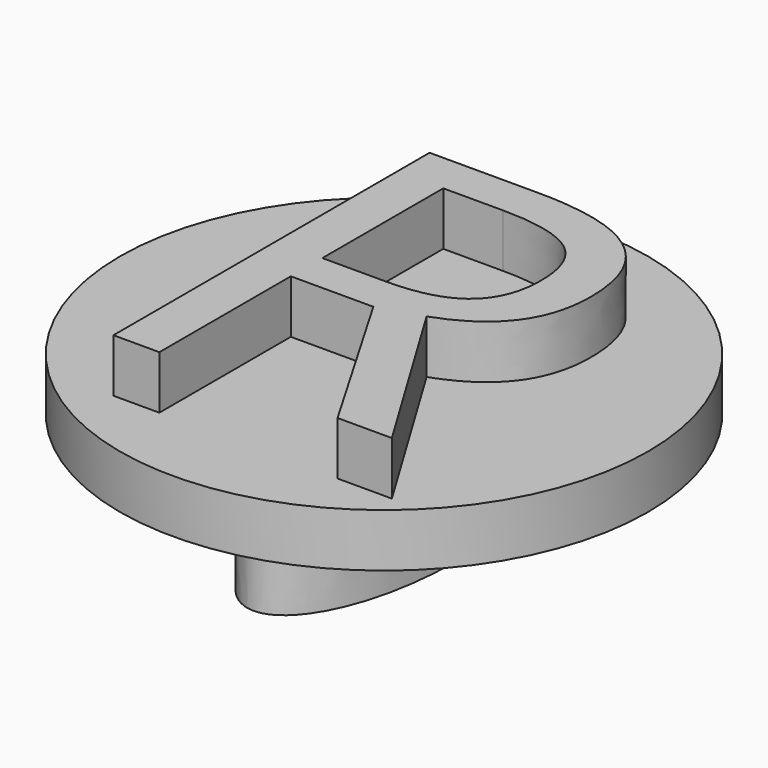
from build123d import *

# Parameters (mm, degrees)
F0_TEXT_SIZE = 26.3821948061
F1_DEPTH     = 5.08
F2_R         = 12.5880099823
F3_DEPTH     = 2.54
F5_DEPTH     = 5.08


# Not quite as in the source:
# - Text() gives the source's letters only with a copy of the font that has no kerning and outlines rounded to 1/6400 em; it was checked with that copy


with BuildPart() as f1:
    # F0 (on Top) → F1 (new body)
    with BuildSketch(Plane.XY):
        with Locations((-31.6586345434, -4.8926980235)):
            Text('R', F0_TEXT_SIZE, font='Open Sans', text_align=(TextAlign.LEFT, TextAlign.BOTTOM))
    extrude(amount=F1_DEPTH)

    # F2 (on Top) → F3 (join)
    with BuildSketch(Plane.XY):
        with Locations((-23.3122650534, 4.0292805061)):
            Circle(F2_R)
    extrude(amount=F3_DEPTH)

    # F4 (on face) → F5 (join)
    with BuildSketch(Plane(origin=(0, 0, 0), x_dir=(1, 0, 0), z_dir=(0, 0, -1))):
        with BuildLine():
            add(Edge.make_bspline(
                [(-23.3122650534, 3.7414748222), (-29.1932017859, 3.7414748222), (-26.2527334196, -7.9146581702), (-23.3122650534, -19.5707911626), (-20.3717966871, -7.9146581702), (-17.4313283209, 3.7414748222), (-23.3122650534, 3.7414748222)],
                knots=[0, 0, 0, 2.0943951024, 2.0943951024, 4.1887902048, 4.1887902048, 6.2831853072, 6.2831853072, 6.2831853072], degree=2, weights=[1, 0.5, 1, 0.5, 1, 0.5, 1]))
        make_face()
    extrude(amount=F5_DEPTH)


solid = f1.part
